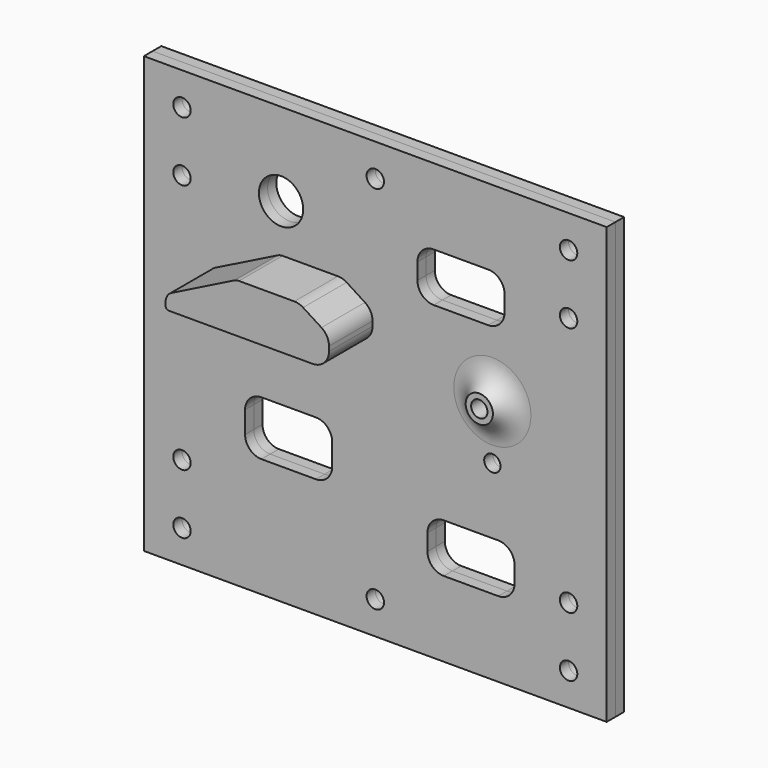
from build123d import *

# Parameters (mm, degrees)
F0_R          = 2.5
F0_R_2        = 1.6
F0_R_3        = 1.5
F1_DEPTH      = 2
F3_DEPTH      = 10
F4_DEPTH      = 3
F4_DEPTH_BACK = 2
F6_R          = 4.0661391715
F7_DEPTH      = 25


# Not quite as in the source:
# - a fillet or chamfer that OpenCascade refuses, or shapes differently, is made with other operations: its cross-section is extruded or revolved along the edge and cut away or added


with BuildPart() as f1:
    # F0 (on Front) → F1 (new body)
    with BuildSketch(Plane.XZ):
        Polygon((42.5, -4), (42.5, 4), (42.5, 6), (-42.5, 6), (-42.5, 4), (-42.5, -4), (-42.5, -34), (42.5, -34), align=None)
        with BuildLine():
            Line((-3.5, -27), (-29.945935972, -27))
            ThreePointArc((-29.945935972, -27), (-30.3377184034, -26.8377184034), (-30.5, -26.445935972))
            Line((-30.5, -26.445935972), (-30.5, -25.7360679775))
            ThreePointArc((-30.5, -25.7360679775), (-30.2013016167, -24.6846057533), (-29.394427191, -23.9472135955))
            Line((-29.394427191, -23.9472135955), (-17.922291236, -18.211145618))
            ThreePointArc((-17.922291236, -18.211145618), (-17.4873698861, -18.0535020211), (-17.027864045, -18))
            Line((-17.027864045, -18), (-6.8736020616, -18))
            ThreePointArc((-6.8736020616, -18), (-6.0348391003, -18.1196394853), (-5.262975585, -18.4690155368))
            Line((-5.262975585, -18.4690155368), (-1.8893735234, -20.6158532124))
            ThreePointArc((-1.8893735234, -20.6158532124), (-0.87018257, -21.7032102011), (-0.5, -23.1468376756))
            Line((-0.5, -23.1468376756), (-0.5, -24))
            ThreePointArc((-0.5, -24), (-1.3786796564, -26.1213203436), (-3.5, -27))
        make_face(mode=Mode.SUBTRACT)
        with Locations((21.5, -29)):
            Circle(F0_R, mode=Mode.SUBTRACT)
        with Locations((-35.5, -11)):
            Circle(F0_R_2, mode=Mode.SUBTRACT)
        with Locations((-35.5, 0)):
            Circle(F0_R_2, mode=Mode.SUBTRACT)
        with Locations((35.5, -11)):
            Circle(F0_R_2, mode=Mode.SUBTRACT)
        Circle(F0_R_2, mode=Mode.SUBTRACT)
        with Locations((35.5, 0)):
            Circle(F0_R_2, mode=Mode.SUBTRACT)
        with BuildLine():
            ThreePointArc((-30.5, -26.445935972), (-30.3377184034, -26.8377184034), (-29.945935972, -27))
            Line((-29.945935972, -27), (-3.5, -27))
            ThreePointArc((-3.5, -27), (-1.3786796564, -26.1213203436), (-0.5, -24))
            Line((-0.5, -24), (-0.5, -23.1468376756))
            ThreePointArc((-0.5, -23.1468376756), (-0.87018257, -21.7032102011), (-1.8893735234, -20.6158532124))
            Line((-1.8893735234, -20.6158532124), (-5.262975585, -18.4690155368))
            ThreePointArc((-5.262975585, -18.4690155368), (-6.0348391003, -18.1196394853), (-6.8736020616, -18))
            Line((-6.8736020616, -18), (-17.027864045, -18))
            ThreePointArc((-17.027864045, -18), (-17.4873698861, -18.0535020211), (-17.922291236, -18.211145618))
            Line((-17.922291236, -18.211145618), (-29.394427191, -23.9472135955))
            ThreePointArc((-29.394427191, -23.9472135955), (-30.2013016167, -24.6846057533), (-30.5, -25.7360679775))
            Line((-30.5, -25.7360679775), (-30.5, -26.445935972))
        make_face()
        with Locations((21.5, -29)):
            Circle(F0_R)
        with Locations((21.5, -29)):
            Circle(F0_R_3, mode=Mode.SUBTRACT)
    extrude(amount=-F1_DEPTH)

    # F2: F1 across face


with BuildPart() as f1_1:
    add(f1.part)
    add(f1.part.mirror(Plane(origin=(0, 1, -34), x_dir=(1, 0, 0), z_dir=(0, 0, -1))))

    # F0 (on Front) → F3 (join)
    with BuildSketch(Plane.XZ):
        with BuildLine():
            ThreePointArc((-30.5, -26.445935972), (-30.3377184034, -26.8377184034), (-29.945935972, -27))
            Line((-29.945935972, -27), (-3.5, -27))
            ThreePointArc((-3.5, -27), (-1.3786796564, -26.1213203436), (-0.5, -24))
            Line((-0.5, -24), (-0.5, -23.1468376756))
            ThreePointArc((-0.5, -23.1468376756), (-0.87018257, -21.7032102011), (-1.8893735234, -20.6158532124))
            Line((-1.8893735234, -20.6158532124), (-5.262975585, -18.4690155368))
            ThreePointArc((-5.262975585, -18.4690155368), (-6.0348391003, -18.1196394853), (-6.8736020616, -18))
            Line((-6.8736020616, -18), (-17.027864045, -18))
            ThreePointArc((-17.027864045, -18), (-17.4873698861, -18.0535020211), (-17.922291236, -18.211145618))
            Line((-17.922291236, -18.211145618), (-29.394427191, -23.9472135955))
            ThreePointArc((-29.394427191, -23.9472135955), (-30.2013016167, -24.6846057533), (-30.5, -25.7360679775))
            Line((-30.5, -25.7360679775), (-30.5, -26.445935972))
        make_face()
    extrude(amount=F3_DEPTH)

    # F0 (on Front) → F4 (join, two sides)
    with BuildSketch(Plane.XZ) as f4_sk:
        with Locations((21.5, -29)):
            Circle(F0_R)
        with Locations((21.5, -29)):
            Circle(F0_R_3, mode=Mode.SUBTRACT)
    extrude(amount=F4_DEPTH)
    extrude(f4_sk.sketch, amount=-F4_DEPTH_BACK)

    # F5: fillet of radius 5 on 1 edges, made by hand

    # F5_s1 → F5_t2 (revolve)
    with BuildSketch(Plane.XY.offset(-29)):
        with BuildLine():
            ThreePointArc((28.582575695, 0), (25.8439629074, -0.8166998673), (24, -3))
            Line((24, -3), (24, 0))
            Line((24, 0), (28.582575695, 0))
        make_face()
    revolve(axis=Axis((21.5, 0, -29), (0, -1, 0)))

    # F6 (on face) → F7 (cut)
    with BuildSketch(Plane.XZ):
        with BuildLine():
            Line((22.5772393979, -51.1348243654), (12.5772393979, -51.1348243654))
            ThreePointArc((12.5772393979, -51.1348243654), (10.4559190544, -52.0135040218), (9.5772393979, -54.1348243654))
            Line((9.5772393979, -54.1348243654), (9.5772393979, -57.1348243654))
            ThreePointArc((9.5772393979, -57.1348243654), (10.4559190544, -59.2561447089), (12.5772393979, -60.1348243654))
            Line((12.5772393979, -60.1348243654), (22.5772393979, -60.1348243654))
            ThreePointArc((22.5772393979, -60.1348243654), (24.6985597415, -59.2561447089), (25.5772393979, -57.1348243654))
            Line((25.5772393979, -57.1348243654), (25.5772393979, -54.1348243654))
            ThreePointArc((25.5772393979, -54.1348243654), (24.6985597415, -52.0135040218), (22.5772393979, -51.1348243654))
        make_face()
        with BuildLine():
            Line((-10.9149579704, -42.1334951818), (-20.9149579704, -42.1334951818))
            ThreePointArc((-20.9149579704, -42.1334951818), (-23.0362783139, -43.0121748382), (-23.9149579704, -45.1334951818))
            Line((-23.9149579704, -45.1334951818), (-23.9149579704, -49.1334951818))
            ThreePointArc((-23.9149579704, -49.1334951818), (-23.0362783139, -51.2548155254), (-20.9149579704, -52.1334951818))
            Line((-20.9149579704, -52.1334951818), (-10.9149579704, -52.1334951818))
            ThreePointArc((-10.9149579704, -52.1334951818), (-8.7936376268, -51.2548155254), (-7.9149579704, -49.1334951818))
            Line((-7.9149579704, -49.1334951818), (-7.9149579704, -45.1334951818))
            ThreePointArc((-7.9149579704, -45.1334951818), (-8.7936376268, -43.0121748382), (-10.9149579704, -42.1334951818))
        make_face()
        with BuildLine():
            Line((20.7370246872, -7.9352889061), (10.7370246872, -7.9352889061))
            ThreePointArc((10.7370246872, -7.9352889061), (8.6157043437, -8.8139685625), (7.7370246872, -10.9352889061))
            Line((7.7370246872, -10.9352889061), (7.7370246872, -13.9352889061))
            ThreePointArc((7.7370246872, -13.9352889061), (8.6157043437, -16.0566092497), (10.7370246872, -16.9352889061))
            Line((10.7370246872, -16.9352889061), (20.7370246872, -16.9352889061))
            ThreePointArc((20.7370246872, -16.9352889061), (22.8583450308, -16.0566092497), (23.7370246872, -13.9352889061))
            Line((23.7370246872, -13.9352889061), (23.7370246872, -10.9352889061))
            ThreePointArc((23.7370246872, -10.9352889061), (22.8583450308, -8.8139685625), (20.7370246872, -7.9352889061))
        make_face()
        with Locations((-17.3052940518, -9.25668329)):
            Circle(F6_R)
    extrude(amount=-F7_DEPTH, mode=Mode.SUBTRACT)


with BuildPart() as f8_1:
    # F8: instance of F1
    add(f1_1.part.mirror(Plane(origin=(-0.2442776853, 2, -33.8837241542), x_dir=(-1, 0, 0), z_dir=(0, 1, 0))))


solid = Compound([f1_1.part, f8_1.part])
